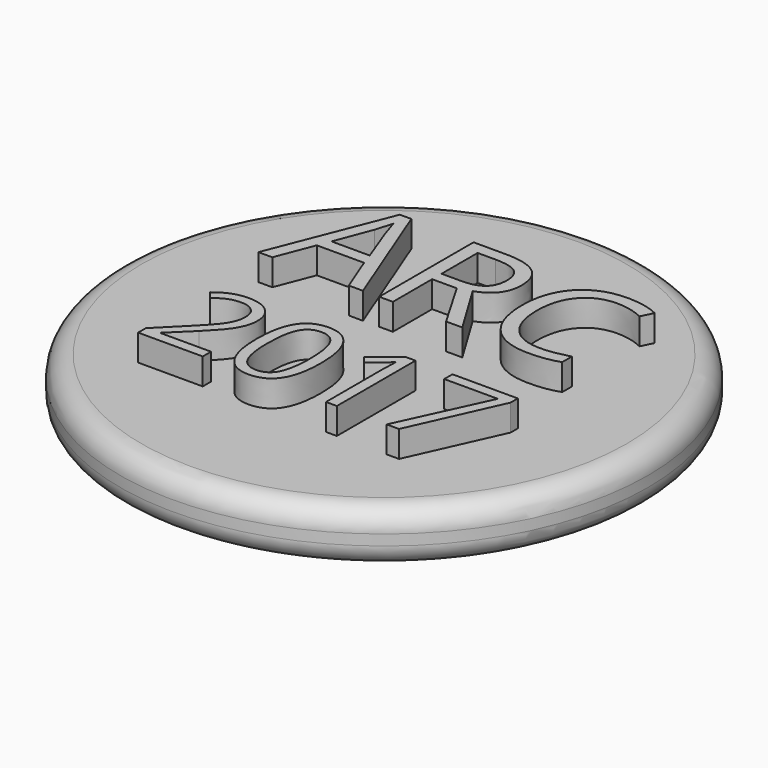
from build123d import *

# Parameters (mm, degrees)
F0_R         = 63.5
F1_DEPTH     = 12.7
F2_TEXT_SIZE = 39.7522008477
F3_DEPTH     = 6.35
F4_TEXT_SIZE = 33.1169360315
F5_DEPTH     = 6.35
F6_R         = 5.08


# Not quite as in the source:
# - Text() gives the source's letters only with a copy of the font that has no kerning and outlines rounded to 1/6400 em; it was checked with that copy


with BuildPart() as f1:
    # F0 (on Top) → F1 (new body)
    with BuildSketch(Plane.XY):
        Circle(F0_R)
    extrude(amount=F1_DEPTH)

    # F2 (on face) → F3 (join)
    with BuildSketch(Plane.XY.offset(12.7)):
        with Locations((-36.696964607, 8.0753767221)):
            Text('ARC', F2_TEXT_SIZE, font='Open Sans', text_align=(TextAlign.LEFT, TextAlign.BOTTOM))
    extrude(amount=F3_DEPTH)

    # F4 (on face) → F5 (join)
    with BuildSketch(Plane.XY.offset(12.7)):
        with Locations((-35.5167912319, -31.5927865769)):
            Text('2017', F4_TEXT_SIZE, font='Open Sans', text_align=(TextAlign.LEFT, TextAlign.BOTTOM))
    extrude(amount=F5_DEPTH)

    # F6
    f6_edges = [f1.edges().sort_by_distance(p)[0] for p in [
        (63.5, 0, 6.35),
        (-63.5, 0, 0),
        (-63.5, 0, 12.7),
    ]]
    fillet(f6_edges, radius=F6_R)


solid = f1.part
